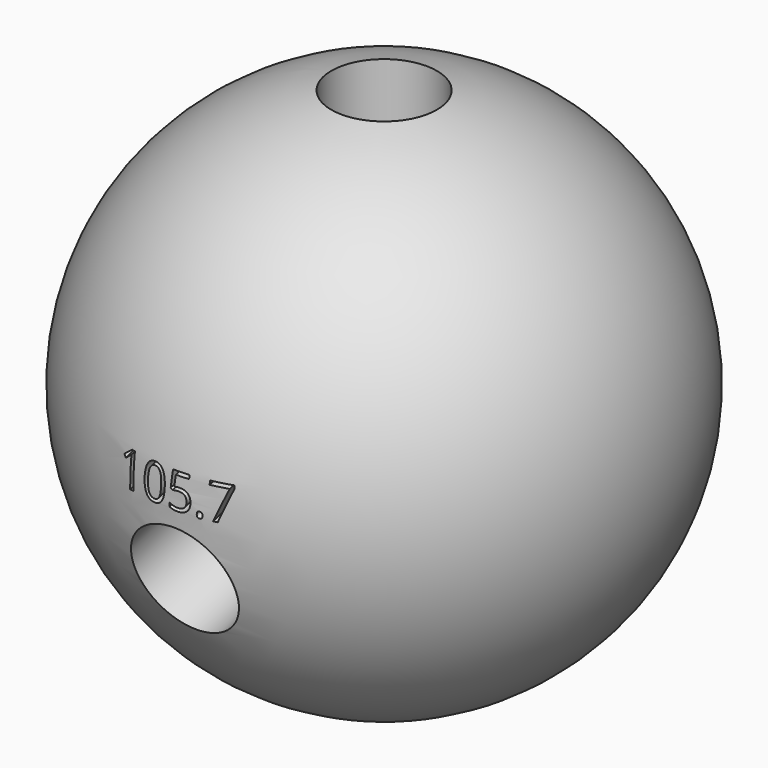
from build123d import *

# Parameters (mm, degrees)
F4_R         = 3.175
F5_DEPTH     = 50.8
F7_ANGLE     = 105.7
F9_TEXT_SIZE = 2.73034287
F10_DEPTH    = 6.35


# Not quite as in the source:
# - a length typed as a fraction of an inch, garbled in the dataset ("3 / 203.2 mm" for 3/8 in), is restored
# - Text() gives the source's letters only with a copy of the font that has no kerning and outlines rounded to 1/6400 em; it was checked with that copy


with BuildPart() as f2:
    # F0 (on Front) → F2 (revolve)
    with BuildSketch(Plane.XZ):
        with BuildLine():
            Line((0, -15.875), (0, 15.875))
            ThreePointArc((0, 15.875), (-15.875, 0), (0, -15.875))
        make_face()
    revolve(axis=Axis((0, 0, 0), (0, 0, 1)))

    # F9 (on offset) → F10 (cut)
    with BuildSketch(Plane(origin=(0, -18.3392777694, -5.1549384958), x_dir=(1, 0, 0), z_dir=(0, -0.9626917464, -0.270600446))):
        with Locations((-3.5044377352, 4.1143381968)):
            Text('105.7', F9_TEXT_SIZE, font='Open Sans', text_align=(TextAlign.LEFT, TextAlign.BOTTOM))
    extrude(amount=-F10_DEPTH, mode=Mode.SUBTRACT)


with BuildPart() as f5:
    # F4 (on offset) → F5 (new body)
    with BuildSketch(Plane.XY.offset(6.35)):
        Circle(F4_R)
    extrude(amount=F5_DEPTH)


with BuildPart() as f7_1:
    # F7: copy of F5
    add(f5.part.rotate(Axis((29.0340390056, 0, 0), (1, 0, 0)), F7_ANGLE))


with BuildPart() as f2_1:
    add(f2.part)

    # F11: cut F5, F7_1
    add(f5.part, mode=Mode.SUBTRACT)
    add(f7_1.part, mode=Mode.SUBTRACT)


solid = f2_1.part
